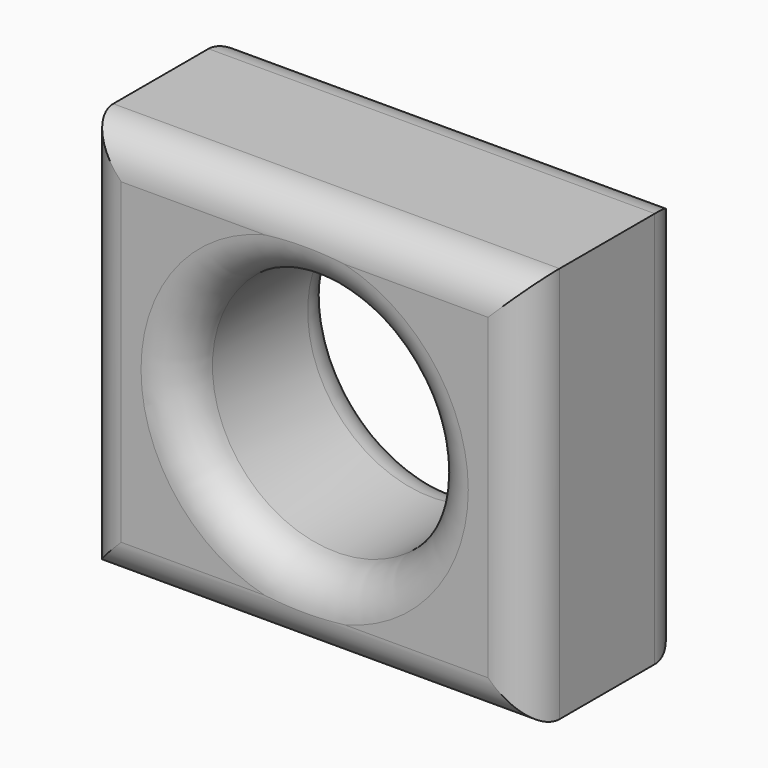
from build123d import *

# Parameters (mm, degrees)
F0_W        = 57.15
F0_H        = 50.8
F1_DEPTH    = 25.4
F2_DEPTH    = 25.4
F3_DEPTH    = 25.4
F4_R        = 15.875
F5_DEPTH    = 25.4
F6_T1_DEPTH = 82.55
F6_T3_DEPTH = 76.2
F7_T1_DEPTH = 82.55
F7_T3_DEPTH = 76.2


# Not quite as in the source:
# - a fillet or chamfer that OpenCascade refuses, or shapes differently, is made with other operations: its cross-section is extruded or revolved along the edge and cut away or added


with BuildPart() as f1:
    # F0 (on Front) → F1 (new body)
    with BuildSketch(Plane.XZ):
        with Locations((28.575, -25.4)):
            Rectangle(F0_W, F0_H)
    extrude(amount=F1_DEPTH)

    # F0 (on Front) → F2 (join)
    with BuildSketch(Plane.XZ):
        with Locations((28.575, -25.4)):
            Rectangle(F0_W, F0_H)
    extrude(amount=F2_DEPTH)

    # F0 (on Front) → F3 (join)
    with BuildSketch(Plane.XZ):
        with Locations((28.575, -25.4)):
            Rectangle(F0_W, F0_H)
    extrude(amount=F3_DEPTH)

    # F4 (on face) → F5 (cut)
    with BuildSketch(Plane.XZ.offset(25.4)):
        with Locations((28.575, -25.4)):
            Circle(F4_R)
    extrude(amount=-F5_DEPTH, mode=Mode.SUBTRACT)

    # F6: fillet of radius 5.08 on 5 edges, made by hand

    # F6_s2 → F6_t1 (cut)
    with BuildSketch(Plane.YZ.offset(-12.7)):
        with BuildLine():
            ThreePointArc((-20.32, 0), (-23.9121024484, -1.4878975516), (-25.4, -5.08))
            Line((-25.4, -5.08), (-25.4, 0))
            Line((-25.4, 0), (-20.32, 0))
        make_face()
        with BuildLine():
            ThreePointArc((-25.4, -45.72), (-23.9121024484, -49.3121024484), (-20.32, -50.8))
            Line((-20.32, -50.8), (-25.4, -50.8))
            Line((-25.4, -50.8), (-25.4, -45.72))
        make_face()
    extrude(amount=F6_T1_DEPTH, mode=Mode.SUBTRACT)

    # F6_s4 → F6_t3 (cut)
    with BuildSketch(Plane.XY.offset(-63.5)):
        with BuildLine():
            ThreePointArc((57.15, -20.32), (55.6621024484, -23.9121024484), (52.07, -25.4))
            Line((52.07, -25.4), (57.15, -25.4))
            Line((57.15, -25.4), (57.15, -20.32))
        make_face()
        with BuildLine():
            ThreePointArc((0, -20.32), (1.4878975516, -23.9121024484), (5.08, -25.4))
            Line((5.08, -25.4), (0, -25.4))
            Line((0, -25.4), (0, -20.32))
        make_face()
    extrude(amount=F6_T3_DEPTH, mode=Mode.SUBTRACT)

    # F6_s5 → F6_t6 (revolve, cut)
    with BuildSketch(Plane.XY.offset(-25.4)):
        with BuildLine():
            ThreePointArc((49.53, -25.4), (45.9378975516, -23.9121024484), (44.45, -20.32))
            Line((44.45, -20.32), (44.45, -25.4))
            Line((44.45, -25.4), (49.53, -25.4))
        make_face()
    revolve(axis=Axis((28.575, -25.4, -25.4), (0, -1, 0)), mode=Mode.SUBTRACT)

    # F7: fillet of radius 5.08 on 5 edges, made by hand

    # F7_s2 → F7_t1 (cut)
    with BuildSketch(Plane.YZ.offset(-12.7)):
        with BuildLine():
            ThreePointArc((-5.08, 0), (-1.4878975516, -1.4878975516), (0, -5.08))
            Line((0, -5.08), (0, 0))
            Line((0, 0), (-5.08, 0))
        make_face()
        with BuildLine():
            ThreePointArc((0, -45.72), (-1.4878975516, -49.3121024484), (-5.08, -50.8))
            Line((-5.08, -50.8), (0, -50.8))
            Line((0, -50.8), (0, -45.72))
        make_face()
    extrude(amount=F7_T1_DEPTH, mode=Mode.SUBTRACT)

    # F7_s4 → F7_t3 (cut)
    with BuildSketch(Plane.XY.offset(-63.5)):
        with BuildLine():
            ThreePointArc((52.07, 0), (55.6621024484, -1.4878975516), (57.15, -5.08))
            Line((57.15, -5.08), (57.15, 0))
            Line((57.15, 0), (52.07, 0))
        make_face()
        with BuildLine():
            ThreePointArc((5.08, 0), (1.4878975516, -1.4878975516), (0, -5.08))
            Line((0, -5.08), (0, 0))
            Line((0, 0), (5.08, 0))
        make_face()
    extrude(amount=F7_T3_DEPTH, mode=Mode.SUBTRACT)

    # F7_s5 → F7_t6 (revolve, cut)
    with BuildSketch(Plane.XY.offset(-25.4)):
        with BuildLine():
            ThreePointArc((49.53, 0), (45.9378975516, -1.4878975516), (44.45, -5.08))
            Line((44.45, -5.08), (44.45, 0))
            Line((44.45, 0), (49.53, 0))
        make_face()
    revolve(axis=Axis((28.575, 0, -25.4), (0, -1, 0)), mode=Mode.SUBTRACT)


solid = f1.part
